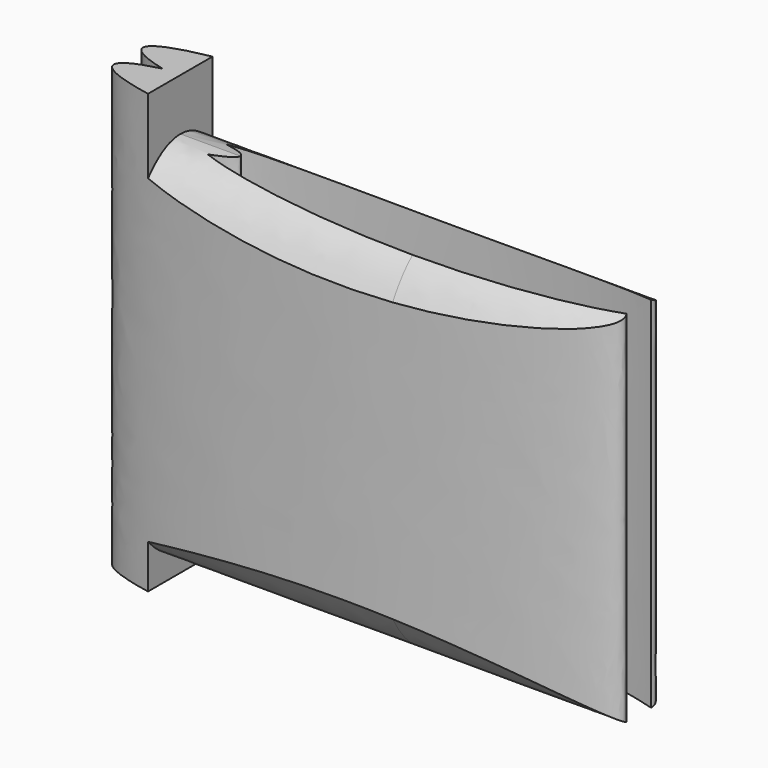
from build123d import *

# Parameters (mm, degrees)
F1_DEPTH = 60
F3_W     = 77.2900707926
F3_H     = 78.8167894955
F4_DEPTH = 35


# Not quite as in the source:
# - a feature names something its author has since deleted; it is built from what else it names


with BuildPart() as f1:
    # F0 (on Top) → F1 (new body)
    with BuildSketch(Plane.XY):
        with BuildLine():
            add(Edge.make_bspline(
                [(-30.0608685873, -1.5203571292), (-5.6405426455, -8.834452637), (27.7624027295, -2.0795957538)],
                knots=[0.3898928212, 0.3898928212, 0.3898928212, 2.5948600146, 2.5948600146, 2.5948600146], degree=2, weights=[1, 0.4513813251, 1]))
            add(Edge.make_bspline(
                [(-30.0608685873, -1.5203571292), (-29.7258919475, -1.444990307), (-29.4243618349, -1.3685535103)],
                knots=[5.9128696013, 5.9128696013, 5.9128696013, 5.9513550051, 5.9513550051, 5.9513550051], degree=2, weights=[1, 0.9998148649, 1]))
            add(Edge.make_bspline(
                [(-29.4243618349, -1.3685535103), (-24.0778942029, -0.013243237), (-29.331680365, 1.3448295191)],
                knots=[5.9513550051, 5.9513550051, 5.9513550051, 6.6090485374, 6.6090485374, 6.6090485374], degree=2, weights=[1, 0.9464154117, 1]))
            add(Edge.make_bspline(
                [(-29.331680365, 1.3448295191), (-29.6739386423, 1.4333012665), (-30.0608685873, 1.5203571292)],
                knots=[0.3258632302, 0.3258632302, 0.3258632302, 0.3703157059, 0.3703157059, 0.3703157059], degree=2, weights=[1, 0.9997530073, 1]))
            add(Edge.make_bspline(
                [(27.7807547125, 2.0758800074), (-5.6075522439, 8.8443335431), (-30.0608685873, 1.5203571292)],
                knots=[3.6872381942, 3.6872381942, 3.6872381942, 5.893292486, 5.893292486, 5.893292486], degree=2, weights=[1, 0.4508962326, 1]))
            add(Edge.make_bspline(
                [(27.7807547125, 2.0758800074), (31.6525304456, 8.8517261101), (-14.7779584398, 7.3609874961), (-61.2084473252, 5.8702488821), (-37.4141041042, -0.0173241738)],
                knots=[3.0601434644, 3.0601434644, 3.0601434644, 4.9334637736, 4.9334637736, 6.8067840828, 6.8067840828, 6.8067840828], degree=2, weights=[1, 0.5924818498, 1, 0.5924818498, 1]))
            add(Edge.make_bspline(
                [(-37.4141041042, -0.0173241738), (-61.2859911602, -5.9240843529), (-14.6719135348, -7.3990159224), (31.9421640907, -8.8739474918), (27.7624027295, -2.0795957538)],
                knots=[5.7595865316, 5.7595865316, 5.7595865316, 7.6360111962, 7.6360111962, 9.5124358608, 9.5124358608, 9.5124358608], degree=2, weights=[1, 0.5912307274, 1, 0.5912307274, 1]))
        make_face()
    extrude(amount=F1_DEPTH)

    # F3 (on Right) → F4 (cut, symmetric)
    with BuildSketch(Plane.YZ):
        with Locations((-5.2480897923, 25.6679380407)):
            Rectangle(F3_W, F3_H)
        with BuildLine():
            add(Edge.make_bspline(
                [(0, 52.9021002352), (-19.8873601783, 52.9021002352), (-9.9436800891, 15.4021002352), (0, -22.0978997648), (9.9436800891, 15.4021002352), (19.8873601783, 52.9021002352), (0, 52.9021002352)],
                knots=[0, 0, 0, 2.0943951024, 2.0943951024, 4.1887902048, 4.1887902048, 6.2831853072, 6.2831853072, 6.2831853072], degree=2, weights=[1, 0.5, 1, 0.5, 1, 0.5, 1]))
        make_face(mode=Mode.SUBTRACT)
    extrude(amount=F4_DEPTH, both=True, mode=Mode.SUBTRACT)


solid = f1.part
